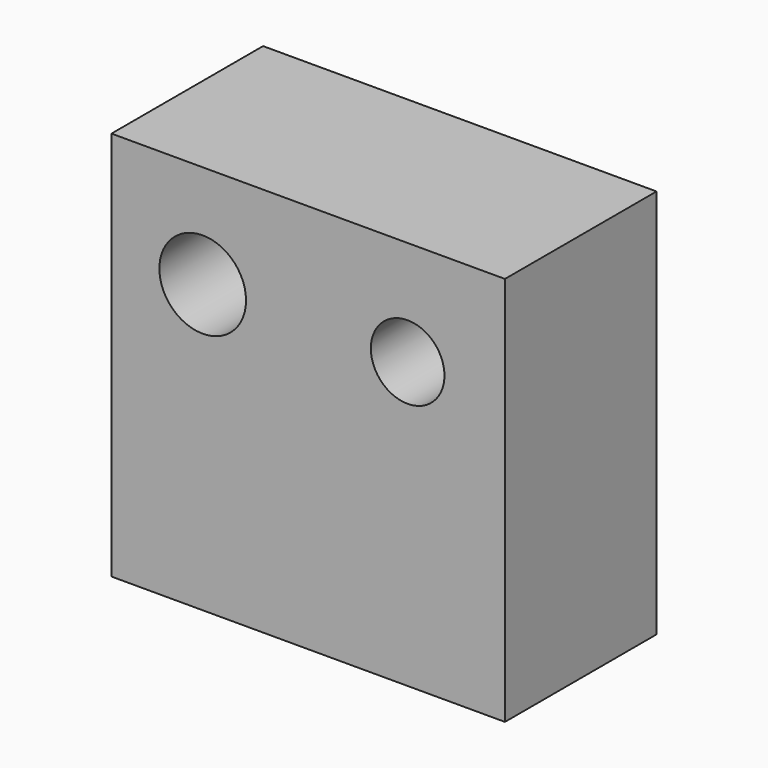
from build123d import *

# Parameters (mm, degrees)
F0_W     = 52.7440756559
F0_H     = 52.2768497467
F1_DEPTH = 25.4
F2_R     = 4.8102139617
F3_DEPTH = 126.0972395539
F4_R     = 4.9351190146
F5_DEPTH = 76.2
F6_R     = 5.8080274439
F8_DEPTH = 25.4


# Not quite as in the source:
# - the program builds the solid bodies; features that only make, move or delete a surface that nothing else refers to are left out


with BuildPart() as f1:
    # F0 (on Front) → F1 (new body)
    with BuildSketch(Plane.XZ):
        with Locations((-1.0988339782, 2.8451383114)):
            Rectangle(F0_W, F0_H)
    extrude(amount=F1_DEPTH)

    # F2 (on Front) → F3 (cut)
    with BuildSketch(Plane.XZ):
        with Locations((-12.8197297454, 11.39511168)):
            Circle(F2_R)
    extrude(amount=-F3_DEPTH, mode=Mode.SUBTRACT)

    # F4 (on face) → F5 (cut)
    with BuildSketch(Plane(origin=(0, 0, 0), x_dir=(-1, 0, 0), z_dir=(0, 1, 0))):
        with Locations((-12.2308423743, 14.9360494688)):
            Circle(F4_R)
    extrude(amount=-F5_DEPTH, mode=Mode.SUBTRACT)

    # F6 (on face) → F8 (cut)
    with BuildSketch(Plane.XZ.offset(25.4)):
        with Locations((-15.2422711253, 15.1493921876)):
            Circle(F6_R)
    extrude(amount=-F8_DEPTH, mode=Mode.SUBTRACT)


solid = f1.part
